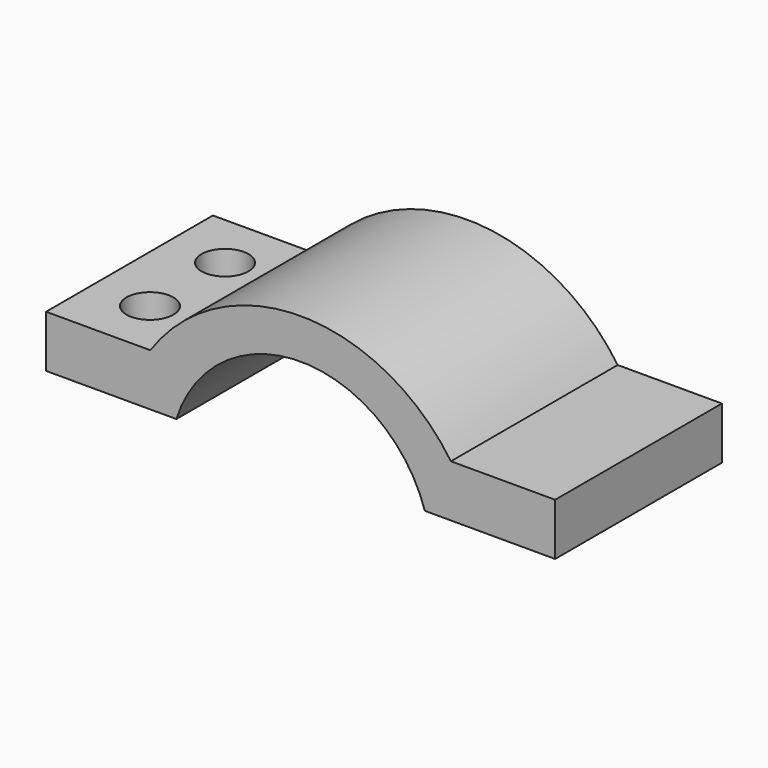
from build123d import *

# Parameters (mm, degrees)
F1_DEPTH = 101.6
F3_D     = 22.86


# Not quite as in the source:
# - a feature names something its author has since deleted; it is built from what else it names
# - the program builds the solid bodies; features that only make, move or delete a surface that nothing else refers to are left out


with BuildPart() as f1:
    # F0 (on Front) → F1 (new body)
    with BuildSketch(Plane.XZ):
        with BuildLine():
            Line((-132.1375894797, -18.6150499344), (-132.1375894797, -44.0150499344))
            Line((-132.1375894797, -44.0150499344), (-68.6375894797, -44.0150499344))
            ThreePointArc((-68.6375894797, -44.0150499344), (-8.0905175805, 0.345930121), (52.4565543186, -44.0150499344))
            Line((52.4565543186, -44.0150499344), (115.9565543186, -44.0150499344))
            Line((115.9565543186, -44.0150499344), (115.9565543186, -18.6150499344))
            Line((115.9565543186, -18.6150499344), (65.1565543186, -18.6150499344))
            ThreePointArc((65.1565543186, -18.6150499344), (-8.0905175805, 19.9056243635), (-81.3375894797, -18.6150499344))
            Line((-81.3375894797, -18.6150499344), (-132.1375894797, -18.6150499344))
        make_face()
    extrude(amount=F1_DEPTH)

    # F3 (through all)
    with Locations(Plane.XY.offset(-18.6150499344)):
        with Locations((-104.1975894797, -27.5148972869), (-104.1975894797, -73.2348972869)):
            Hole(F3_D / 2)


solid = f1.part
